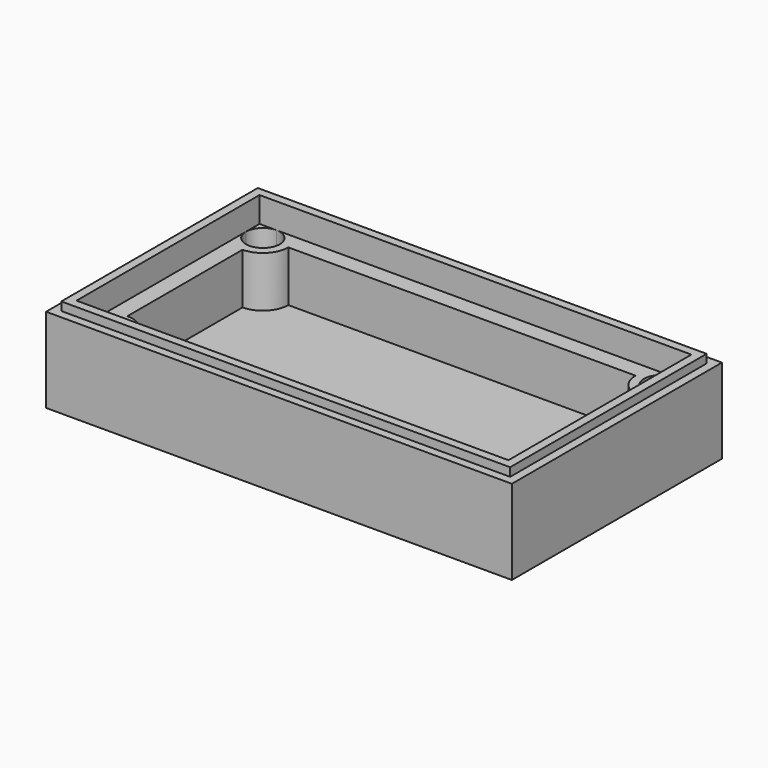
from build123d import *
from build123d import SkipClean  # not in build123d's __all__

# Parameters (mm, degrees)
F0_W      = 55
F0_H      = 31
F2_DEPTH  = 10
F1_W      = 51
F1_H      = 27
F3_DEPTH  = 11
F4_DEPTH  = 8
F5_W      = 51
F5_H      = 2
F6_DEPTH  = 6
F7_W      = 2
F7_H      = 23
F8_DEPTH  = 6
F10_DEPTH = 6
F11_DEPTH = 6


with BuildPart() as f2:
    # F0 (on Top) → F2 (new body)
    with BuildSketch(Plane.XY):
        with Locations((2.9806493223, 1.209073022)):
            Rectangle(F0_W, F0_H)
    extrude(amount=F2_DEPTH)

    # F1 (on face) → F3 (join)
    with BuildSketch(Plane.XY):
        Polygon((-22.5115198195, 15.6954657286), (-23.5115198195, 15.6954657286), (-23.5115198195, -13.3045342714), (29.4884801805, -13.3045342714), (29.4884801805, 15.6954657286), align=None)
        with Locations((2.9884801805, 1.1954657286)):
            Rectangle(F1_W, F1_H, mode=Mode.SUBTRACT)
    extrude(amount=F3_DEPTH)

    # F4 (cut): a face of the model
    f4_faces = [f2.faces().sort_by_distance(p)[0] for p in [
        (2.9884801805, 1.1954657286, 10),
    ]]
    extrude(f4_faces, amount=-F4_DEPTH, mode=Mode.SUBTRACT)

    # F5 (on face) → F6 (join)
    with BuildSketch(Plane.XY.offset(2)):
        with Locations((2.9884801805, 13.6954657286)):
            Rectangle(F5_W, F5_H)
        with Locations((2.9884801805, -11.3045342714)):
            Rectangle(F5_W, F5_H)
    extrude(amount=F6_DEPTH)

    # F7 (on face) → F8 (join)
    with BuildSketch(Plane.XY.offset(2)):
        with Locations((27.4884801805, 1.1954657286)):
            Rectangle(F7_W, F7_H)
        with Locations((-21.5115198195, 1.1954657286)):
            Rectangle(F7_W, F7_H)
    extrude(amount=F8_DEPTH)

    # F9 (on face) → F10 (join)
    with BuildSketch(Plane.XY.offset(8)):
        with BuildLine():
            ThreePointArc((-20.5115198195, 9.6954657286), (-18.3901994759, 10.5741453851), (-17.5115198195, 12.6954657286))
            Line((-17.5115198195, 12.6954657286), (-18.5115198195, 12.6954657286))
            ThreePointArc((-18.5115198195, 12.6954657286), (-19.0973062571, 11.2812521663), (-20.5115198195, 10.6954657286))
            Line((-20.5115198195, 10.6954657286), (-20.5115198195, 9.6954657286))
        make_face()
        with BuildLine():
            ThreePointArc((-17.5115198195, -10.3045342714), (-18.3901994759, -8.1832139278), (-20.5115198195, -7.3045342714))
            Line((-20.5115198195, -7.3045342714), (-20.5115198195, -8.3045342714))
            ThreePointArc((-20.5115198195, -8.3045342714), (-19.0973062571, -8.890320709), (-18.5115198195, -10.3045342714))
            Line((-18.5115198195, -10.3045342714), (-17.5115198195, -10.3045342714))
        make_face()
        with BuildLine():
            Line((26.4884801805, -8.3045342714), (26.4884801805, -7.3045342714))
            ThreePointArc((26.4884801805, -7.3045342714), (24.3671598369, -8.1832139278), (23.4884801805, -10.3045342714))
            Line((23.4884801805, -10.3045342714), (24.4884801805, -10.3045342714))
            ThreePointArc((24.4884801805, -10.3045342714), (25.0742666181, -8.890320709), (26.4884801805, -8.3045342714))
        make_face()
        with BuildLine():
            Line((24.4884801805, 12.6954657286), (23.4884801805, 12.6954657286))
            ThreePointArc((23.4884801805, 12.6954657286), (24.3671598369, 10.5741453851), (26.4884801805, 9.6954657286))
            Line((26.4884801805, 9.6954657286), (26.4884801805, 10.6954657286))
            ThreePointArc((26.4884801805, 10.6954657286), (25.0742666181, 11.2812521663), (24.4884801805, 12.6954657286))
        make_face()
    extrude(amount=-F10_DEPTH)

    # F9 (on face) → F11 (cut)
    with BuildSketch(Plane.XY.offset(8)):
        with BuildLine():
            Line((-20.5115198195, 12.6954657286), (-18.5115198195, 12.6954657286))
            ThreePointArc((-18.5115198195, 12.6954657286), (-19.0973062461, 14.10967928), (-20.5115197883, 14.6954657286))
            ThreePointArc((-20.5115197883, 14.6954657286), (-21.9257333708, 14.1096793021), (-22.5115198195, 12.6954657286))
            ThreePointArc((-22.5115198195, 12.6954657286), (-21.9257333819, 11.2812521663), (-20.5115198195, 10.6954657286))
            Line((-20.5115198195, 10.6954657286), (-20.5115198195, 12.6954657286))
        make_face()
        with BuildLine():
            Line((-20.5115198195, -10.3045342714), (-20.5115198195, -8.3045342714))
            ThreePointArc((-20.5115198195, -8.3045342714), (-21.9257333819, -8.890320709), (-22.5115198195, -10.3045342714))
            ThreePointArc((-22.5115198195, -10.3045342714), (-21.9257333819, -11.7187478337), (-20.5115198195, -12.3045342714))
            ThreePointArc((-20.5115198195, -12.3045342714), (-19.0973062571, -11.7187478337), (-18.5115198195, -10.3045342714))
            Line((-18.5115198195, -10.3045342714), (-20.5115198195, -10.3045342714))
        make_face()
        with BuildLine():
            ThreePointArc((28.4884801805, -10.3045342714), (27.9026937429, -8.890320709), (26.4884801805, -8.3045342714))
            Line((26.4884801805, -8.3045342714), (26.4884801805, -10.3045342714))
            Line((26.4884801805, -10.3045342714), (24.4884801805, -10.3045342714))
            ThreePointArc((24.4884801805, -10.3045342714), (25.0742666181, -11.7187478337), (26.4884801805, -12.3045342714))
            ThreePointArc((26.4884801805, -12.3045342714), (27.9026937429, -11.7187478337), (28.4884801805, -10.3045342714))
        make_face()
        with BuildLine():
            ThreePointArc((26.4884801805, 14.6954657286), (25.0742666181, 14.109679291), (24.4884801805, 12.6954657286))
            Line((24.4884801805, 12.6954657286), (26.4884801805, 12.6954657286))
            Line((26.4884801805, 12.6954657286), (26.4884801805, 10.6954657286))
            ThreePointArc((26.4884801805, 10.6954657286), (27.9026937429, 11.2812521663), (28.4884801805, 12.6954657286))
            ThreePointArc((28.4884801805, 12.6954657286), (27.9026937429, 14.109679291), (26.4884801805, 14.6954657286))
        make_face()
    with SkipClean():  # cleaning this boolean's faces spoils the solid; the shape is the same uncleaned
        extrude(amount=-F11_DEPTH, mode=Mode.SUBTRACT)


solid = f2.part
